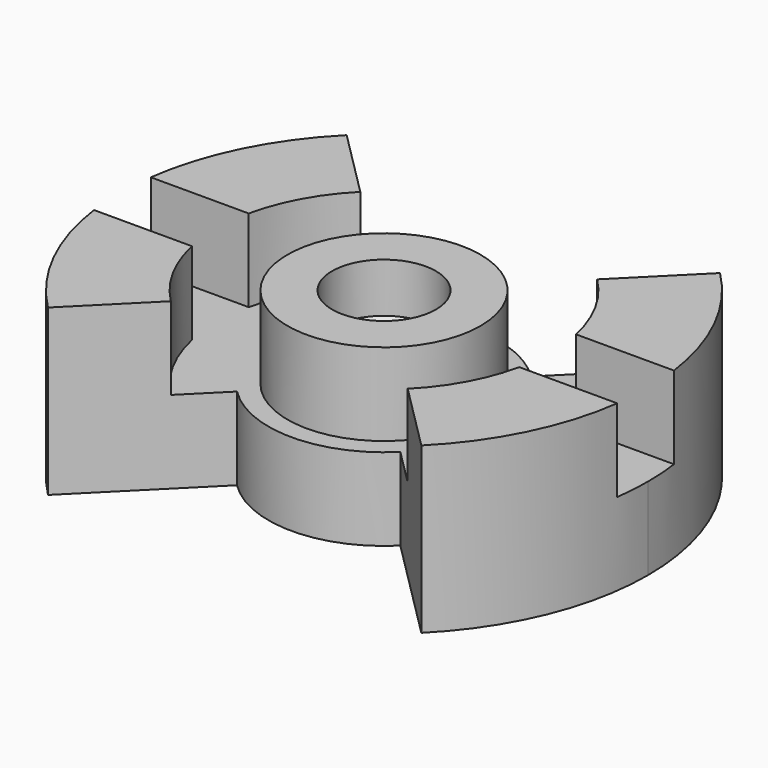
from build123d import *

# Parameters (mm, degrees)
F0_R     = 3.07975
F1_DEPTH = 6.35
F2_R     = 3.71475
F2_R_2   = 2.00025
F3_DEPTH = 3.175
F4_SIZE  = 1.27


# Not quite as in the source:
# - a feature names something its author has since deleted; it is built from what else it names


with BuildPart() as f1:
    # F0 (on Top) → F1 (new body)
    with BuildSketch(Plane.XY):
        with BuildLine():
            ThreePointArc((-4.445, 0), (-4.106644522, 1.7010278569), (-3.1430896424, 3.1430896424))
            Line((-3.1430896424, 3.1430896424), (-7.1842048969, 7.1842048969))
            ThreePointArc((-7.1842048969, 7.1842048969), (-9.3866160503, 3.8880636728), (-10.16, 0))
            ThreePointArc((-10.16, 0), (-9.3866160503, -3.8880636728), (-7.1842048969, -7.1842048969))
            Line((-7.1842048969, -7.1842048969), (-3.1430896424, -3.1430896424))
            ThreePointArc((-3.1430896424, -3.1430896424), (-4.106644522, -1.7010278569), (-4.445, 0))
        make_face()
        with BuildLine():
            ThreePointArc((3.1430896424, -3.1430896424), (4.106644522, -1.7010278569), (4.445, 0))
            ThreePointArc((4.445, 0), (4.106644522, 1.7010278569), (3.1430896424, 3.1430896424))
            ThreePointArc((3.1430896424, 3.1430896424), (0, 4.445), (-3.1430896424, 3.1430896424))
            ThreePointArc((-3.1430896424, 3.1430896424), (-4.106644522, 1.7010278569), (-4.445, 0))
            ThreePointArc((-4.445, 0), (-4.106644522, -1.7010278569), (-3.1430896424, -3.1430896424))
            ThreePointArc((-3.1430896424, -3.1430896424), (0, -4.445), (3.1430896424, -3.1430896424))
        make_face()
        Circle(F0_R, mode=Mode.SUBTRACT)
        with BuildLine():
            ThreePointArc((3.1430896424, 3.1430896424), (4.106644522, 1.7010278569), (4.445, 0))
            ThreePointArc((4.445, 0), (4.106644522, -1.7010278569), (3.1430896424, -3.1430896424))
            Line((3.1430896424, -3.1430896424), (7.1842048969, -7.1842048969))
            ThreePointArc((7.1842048969, -7.1842048969), (9.3866160503, -3.8880636728), (10.16, 0))
            ThreePointArc((10.16, 0), (9.3866160503, 3.8880636728), (7.1842048969, 7.1842048969))
            Line((7.1842048969, 7.1842048969), (3.1430896424, 3.1430896424))
        make_face()
        Circle(F0_R)
    extrude(amount=F1_DEPTH)

    # F2 (on face) → F3 (cut)
    with BuildSketch(Plane.XY.offset(6.35)):
        with BuildLine():
            ThreePointArc((6.298995158, -1.36525), (6.4085819845, -0.6865307789), (6.44525, 0))
            ThreePointArc((6.44525, 0), (6.4085819845, 0.6865307789), (6.298995158, 1.36525))
            ThreePointArc((6.298995158, 1.36525), (5.658033773, 3.0867298855), (4.5574799814, 4.5574799814))
            Line((4.5574799814, 4.5574799814), (3.1430896424, 3.1430896424))
            ThreePointArc((3.1430896424, 3.1430896424), (0, 4.445), (-3.1430896424, 3.1430896424))
            Line((-3.1430896424, 3.1430896424), (-4.5574799814, 4.5574799814))
            ThreePointArc((-4.5574799814, 4.5574799814), (-5.658033773, 3.0867298855), (-6.298995158, 1.36525))
            ThreePointArc((-6.298995158, 1.36525), (-6.44525, 0), (-6.298995158, -1.36525))
            ThreePointArc((-6.298995158, -1.36525), (-5.658033773, -3.0867298855), (-4.5574799814, -4.5574799814))
            Line((-4.5574799814, -4.5574799814), (-3.1430896424, -3.1430896424))
            ThreePointArc((-3.1430896424, -3.1430896424), (0, -4.445), (3.1430896424, -3.1430896424))
            Line((3.1430896424, -3.1430896424), (4.5574799814, -4.5574799814))
            ThreePointArc((4.5574799814, -4.5574799814), (5.658033773, -3.0867298855), (6.298995158, -1.36525))
        make_face()
        Circle(F2_R, mode=Mode.SUBTRACT)
        with BuildLine():
            ThreePointArc((6.298995158, 1.36525), (6.4085819845, 0.6865307789), (6.44525, 0))
            ThreePointArc((6.44525, 0), (6.4085819845, -0.6865307789), (6.298995158, -1.36525))
            Line((6.298995158, -1.36525), (10.0678544108, -1.36525))
            ThreePointArc((10.0678544108, -1.36525), (10.16, 0), (10.0678544108, 1.36525))
            Line((10.0678544108, 1.36525), (6.298995158, 1.36525))
        make_face()
        with BuildLine():
            ThreePointArc((-6.298995158, -1.36525), (-6.44525, 0), (-6.298995158, 1.36525))
            Line((-6.298995158, 1.36525), (-10.0678544108, 1.36525))
            ThreePointArc((-10.0678544108, 1.36525), (-10.16, 0), (-10.0678544108, -1.36525))
            Line((-10.0678544108, -1.36525), (-6.298995158, -1.36525))
        make_face()
        Circle(F2_R_2)
    extrude(amount=-F3_DEPTH, mode=Mode.SUBTRACT)

    # F4
    f4_edges = [f1.edges().sort_by_distance(p)[0] for p in [
        (-2.00025, 0, 3.175),
    ]]
    chamfer(f4_edges, length=F4_SIZE)


solid = f1.part
